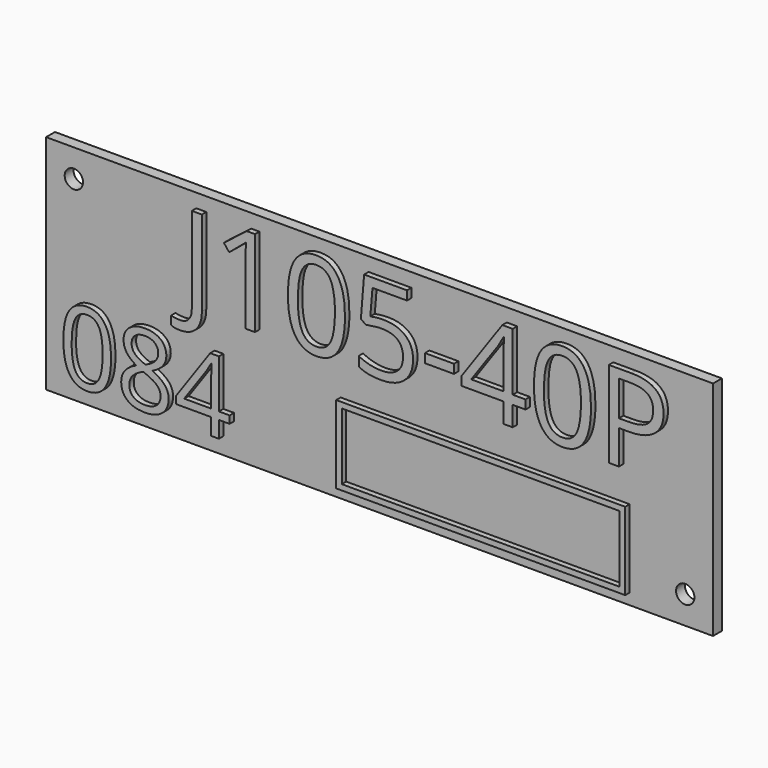
from build123d import *

# Parameters (mm, degrees)
F0_W         = 120
F0_H         = 40
F1_DEPTH     = 2
F3_D         = 3.3
F4_TEXT_SIZE = 21.733388673
F5_DEPTH     = 1
F6_TEXT_SIZE = 18.1818181818
F7_DEPTH     = 1
F8_W         = 52
F8_H         = 14
F8_W_2       = 49.99999962
F8_H_2       = 11.99999962
F9_DEPTH     = 1


# Not quite as in the source:
# - Text() gives the source's letters only with a copy of the font that has no kerning and outlines rounded to 1/6400 em; it was checked with that copy


with BuildPart() as f1:
    # F0 (on Front) → F1 (new body)
    with BuildSketch(Plane.XZ):
        Rectangle(F0_W, F0_H)
    extrude(amount=F1_DEPTH)

    # F3 (through all)
    with Locations(Plane.XZ.offset(2)):
        with Locations((-55, 15), (55, -15)):
            Hole(F3_D / 2)

    # F4 (on face) → F5 (join)
    with BuildSketch(Plane.XZ.offset(2)):
        with Locations((-35, 2)):
            Text('J105-40P', F4_TEXT_SIZE, font='Open Sans', text_align=(TextAlign.LEFT, TextAlign.BOTTOM))
    extrude(amount=F5_DEPTH)

    # F6 (on face) → F7 (join)
    with BuildSketch(Plane.XZ.offset(2)):
        with Locations((-57, -17)):
            Text('084', F6_TEXT_SIZE, font='Open Sans', text_align=(TextAlign.LEFT, TextAlign.BOTTOM))
    extrude(amount=F7_DEPTH)

    # F8 (on face) → F9 (join)
    with BuildSketch(Plane.XZ.offset(2)):
        with Locations((19, -11)):
            Rectangle(F8_W, F8_H)
        with Locations((19, -11)):
            Rectangle(F8_W_2, F8_H_2, mode=Mode.SUBTRACT)
    extrude(amount=F9_DEPTH)


solid = f1.part
